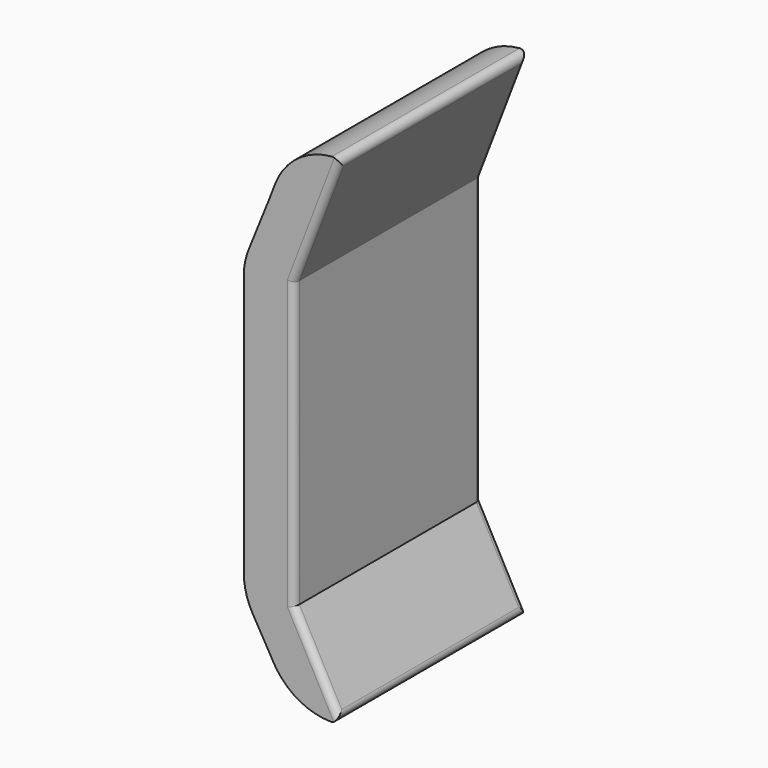
from build123d import *

# Parameters (mm, degrees)
F0_W        = 70
F0_H        = 120
F1_DEPTH    = 7.5
F3_DEPTH    = 70
F4_T4_DEPTH = 168.5345436458
F5_T4_DEPTH = 142.4389014281
F6_R        = 2
F7_T1_DEPTH = 89.4016367136
F7_T3_DEPTH = 96.7750960728
F7_T5_DEPTH = 138.4048613392
F7_T7_DEPTH = 129.7242953335


# Not quite as in the source:
# - a fillet or chamfer that OpenCascade refuses, or shapes differently, is made with other operations: its cross-section is extruded or revolved along the edge and cut away or added


with BuildPart() as f1:
    # F0 (on Right) → F1 (new body, symmetric)
    with BuildSketch(Plane.YZ):
        Rectangle(F0_W, F0_H)
    extrude(amount=F1_DEPTH, both=True)

    # F2 (on face) → F3 (join)
    with BuildSketch(Plane.XZ.offset(35)):
        Polygon((6.7201238232, 77.1365826446), (-7.5, 40), (7.5, 40), (21.7201238232, 77.1365826446), align=None)
        Polygon((7.5, -45), (-7.5, -45), (6.7201238232, -71.4156786483), (21.7201238232, -71.4156786483), align=None)
    extrude(amount=-F3_DEPTH)

    # F4: chamfer of 19 x 7.661 on 1 edges, made by hand


with BuildPart() as f4_tool2:
    # F4_s3 → F4_t4 (new body)
    with BuildSketch(Plane.XZ.offset(-84.2672718229)):
        Polygon((0.161, 60), (-7.5, 41), (-7.5, 60), align=None)
    extrude(amount=F4_T4_DEPTH)

    split(bisect_by=Plane(origin=(-19.8989220202, 0, 7.6195792646), x_dir=(0, 1, 0), z_dir=(-0.933876884, 0, 0.3575946945)), keep=Keep.TOP)


with BuildPart() as f1_1:
    add(f1.part)

    # F4_t1: cut F4_tool2
    add(f4_tool2.part, mode=Mode.SUBTRACT)

    # F5: chamfer of 8.076 x 14 on 1 edges, made by hand


with BuildPart() as f5_tool2:
    # F5_s3 → F5_t4 (new body)
    with BuildSketch(Plane.XZ.offset(71.219450714)):
        Polygon((0.576, -60), (-7.5, -46), (-7.5, -60), align=None)
    extrude(amount=-F5_T4_DEPTH)

    split(bisect_by=Plane(origin=(-24.5966117165, 0, -13.2408812545), x_dir=(0, 1, 0), z_dir=(-0.8805226216, 0, -0.4740041274)), keep=Keep.TOP)


with BuildPart() as f1_2:
    add(f1_1.part)

    # F5_t1: cut F5_tool2
    add(f5_tool2.part, mode=Mode.SUBTRACT)

    # F6
    f6_edges = [f1_2.edges().sort_by_distance(p)[0] for p in [
        (14.610062, -35, 58.568291),
        (7.5, -35, -2.5),
        (14.610062, -35, -58.207839),
        (14.610062, 35, -58.207839),
        (7.5, 35, -2.5),
        (14.610062, 35, 58.568291),
        (21.720124, 0, 77.136583),
        (21.720124, 0, -71.415679),
    ]]
    fillet(f6_edges, radius=F6_R)

    # F7: fillet of radius 20 on 4 edges, made by hand

    # F7_s2 → F7_t1 (cut)
    with BuildSketch(Plane.XZ.offset(-44.7008183568)):
        with BuildLine():
            ThreePointArc((-6.0489277422, 44.5987955748), (-7.1338808548, 40.9289668935), (-7.5, 37.1196726573))
            Line((-7.5, 37.1196726573), (-7.9, 37.1196726573))
            Line((-7.9, 37.1196726573), (-7.9, 41.0776065469))
            Line((-7.9, 41.0776065469), (-6.419906297, 44.7483780332))
            Line((-6.419906297, 44.7483780332), (-6.0489277422, 44.5987955748))
        make_face()
    extrude(amount=F7_T1_DEPTH, mode=Mode.SUBTRACT)

    # F7_s4 → F7_t3 (cut)
    with BuildSketch(Plane.XZ.offset(-48.3875480364)):
        with BuildLine():
            ThreePointArc((-7.5, -40.6449807854), (-6.8194736284, -45.8177884102), (-4.8242061277, -50.6385728345))
            Line((-4.8242061277, -50.6385728345), (-5.1706902503, -50.8384446755))
            Line((-5.1706902503, -50.8384446755), (-7.9, -46.1071003843))
            Line((-7.9, -46.1071003843), (-7.9, -40.6449807854))
            Line((-7.9, -40.6449807854), (-7.5, -40.6449807854))
        make_face()
    extrude(amount=F7_T3_DEPTH, mode=Mode.SUBTRACT)

    # F7_s6 → F7_t5 (cut)
    with BuildSketch(Plane.XZ.offset(-69.2024306696)):
        with BuildLine():
            ThreePointArc((18.8126855564, 77.1365826446), (8.4827015625, 73.1912821466), (1.8278807245, 64.3602388931))
            Line((1.8278807245, 64.3602388931), (1.4543299709, 64.5032767709))
            Line((1.4543299709, 64.5032767709), (6.3465730696, 77.2796205224))
            Line((6.3465730696, 77.2796205224), (6.7201238232, 77.5365826446))
            ThreePointArc((6.7201238232, 77.5365826446), (12.7664046898, 77.5365826446), (18.7788308995, 77.5351473974))
            Line((18.7788308995, 77.5351473974), (18.8126855564, 77.1365826446))
        make_face()
    extrude(amount=F7_T5_DEPTH, mode=Mode.SUBTRACT)

    # F7_s8 → F7_t7 (cut)
    with BuildSketch(Plane.XZ.offset(-64.8621476667)):
        with BuildLine():
            ThreePointArc((1.0582113239, -60.8979600281), (8.2849802368, -68.5111251687), (18.3721027929, -71.4156786483))
            Line((18.3721027929, -71.4156786483), (18.3661715736, -71.8156346717))
            ThreePointArc((18.3661715736, -71.8156346717), (12.546113308, -71.8156786483), (6.7201238232, -71.8156786483))
            Line((6.7201238232, -71.8156786483), (6.3679147746, -71.6052802993))
            Line((6.3679147746, -71.6052802993), (0.7060022753, -61.0875616791))
            Line((0.7060022753, -61.0875616791), (1.0582113239, -60.8979600281))
        make_face()
    extrude(amount=F7_T7_DEPTH, mode=Mode.SUBTRACT)


solid = f1_2.part
